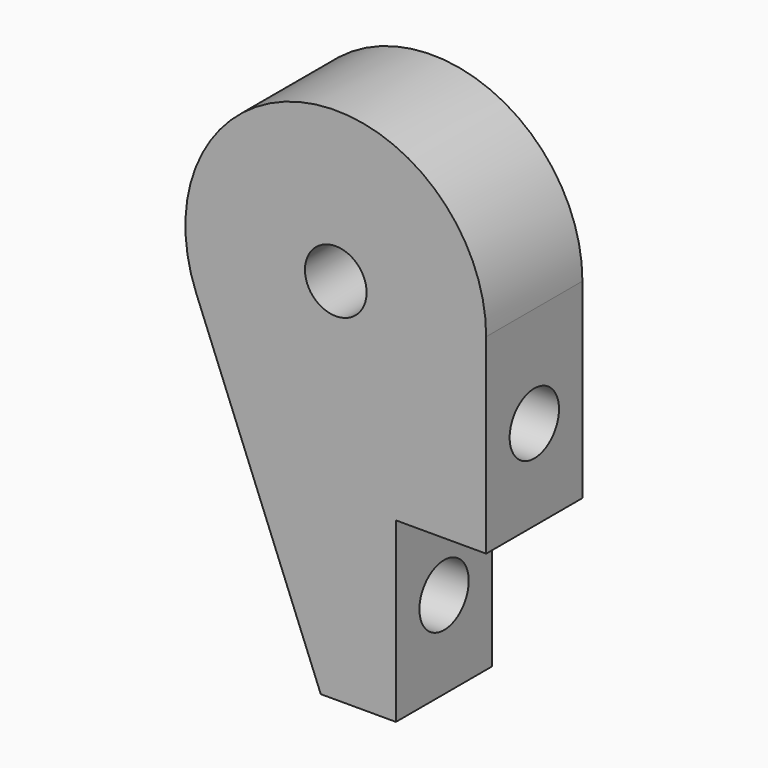
from build123d import *

# Parameters (mm, degrees)
F1_DEPTH = 8
F2_D     = 4.1
F4_D     = 4.1
F4_DEPTH = 12
F4_TIP   = 1.231764269


with BuildPart() as f1:
    # F0 (on Front) → F1 (new body)
    with BuildSketch(Plane.XZ):
        with BuildLine():
            Line((10, -12.7), (10, 0))
            ThreePointArc((10, 0), (-1.8850319079, 9.8207257729), (-9.2893309412, -3.7024762881))
            Line((-9.2893309412, -3.7024762881), (-1, -24.5))
            Line((-1, -24.5), (4, -24.5))
            Line((4, -24.5), (4, -12.7))
            Line((4, -12.7), (10, -12.7))
        make_face()
    extrude(amount=-F1_DEPTH)

    # F2 (through all)
    with Locations(Plane.XZ):
        with Locations((0, 0)):
            Hole(F2_D / 2)

    # F4 (one way)
    with BuildSketch(Plane.YZ.offset(10)):
        with Locations((4, -18.7), (4, -6.7)):
            Circle(F4_D / 2)
    extrude(amount=-F4_DEPTH, mode=Mode.SUBTRACT)
    with Locations(Plane.YZ.offset(10)):
        with Locations((4, -18.7), (4, -6.7)):
            with Locations((0, 0, -(F4_DEPTH + F4_TIP / 2))):  # 118° drill point
                Cone(0, F4_D / 2, F4_TIP, mode=Mode.SUBTRACT)


solid = f1.part
